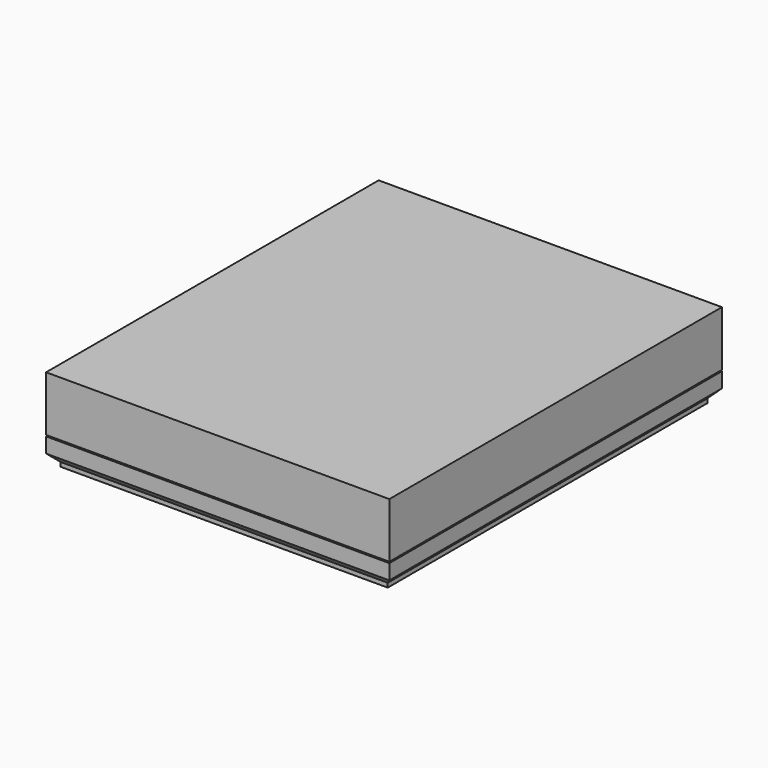
from build123d import *

# Parameters (mm, degrees)
F3_W          = 80.6
F3_H          = 97.6
F4_DEPTH      = 1
F5_W          = 80.6
F5_H          = 97.6
F5_W_2        = 73.6
F5_H_2        = 90.6
F6_DEPTH      = 8.75
F8_DEPTH      = 90.6
F11_W         = 80.6
F11_H         = 97.6
F11_W_2       = 76.8
F11_H_2       = 93.8
F13_DEPTH     = 3.3
F14_W         = 80.6
F14_H         = 97.6
F14_W_2       = 76.8
F14_H_2       = 93.8
F15_DEPTH     = 3
F16_T4_DEPTH  = 76.8
F16_T9_DEPTH  = 93.8
F16_T14_DEPTH = 76.8
F16_T19_DEPTH = 93.8
F16_T25_DEPTH = 81.9433659759
F16_T31_DEPTH = 98.9433659759
F16_T40_DEPTH = 81.9433659759
F16_T46_DEPTH = 98.9433659759
F16_T55_DEPTH = 81.9433659759
F16_T61_DEPTH = 98.9433659759
F16_T70_DEPTH = 98.9433659759
F16_T76_DEPTH = 81.9433659759
F17_W         = 80.6
F17_H         = 97.6
F17_W_2       = 77.4
F17_H_2       = 94.4
F18_DEPTH     = 3.2


# Not quite as in the source:
# - a fillet or chamfer that OpenCascade refuses, or shapes differently, is made with other operations: its cross-section is extruded or revolved along the edge and cut away or added


with BuildPart() as f4:
    # F3 (on Top) → F4 (new body)
    with BuildSketch(Plane.XY):
        Rectangle(F3_W, F3_H)
    extrude(amount=F4_DEPTH)

    # F5 (on face) → F6 (join)
    with BuildSketch(Plane.XY.offset(1)):
        Rectangle(F5_W, F5_H)
        Rectangle(F5_W_2, F5_H_2, mode=Mode.SUBTRACT)
    extrude(amount=F6_DEPTH)

    # F7 (on face) → F8 (join, through all)
    with BuildSketch(Plane.XZ.offset(-45.3)):
        with BuildLine():
            ThreePointArc((-19.9, 9.75), (-28.35, 1.3), (-36.8, 9.75))
            Line((-36.8, 9.75), (-36.8, 1))
            Line((-36.8, 1), (36.8, 1))
            Line((36.8, 1), (36.8, 9.75))
            ThreePointArc((36.8, 9.75), (28.35, 1.3), (19.9, 9.75))
            Line((19.9, 9.75), (17.9, 9.75))
            ThreePointArc((17.9, 9.75), (9.45, 1.3), (1, 9.75))
            Line((1, 9.75), (-1, 9.75))
            ThreePointArc((-1, 9.75), (-9.45, 1.3), (-17.9, 9.75))
            Line((-17.9, 9.75), (-19.9, 9.75))
        make_face()
    extrude(amount=F8_DEPTH)


with BuildPart() as f10_1:
    # F10: instance of F4
    add(f4.part.mirror(Plane.XY.offset(9.85)))

    # F17 (on face) → F18 (join)
    with BuildSketch(Plane(origin=(0, 0, 9.95), x_dir=(1, 0, 0), z_dir=(0, 0, -1))):
        Rectangle(F17_W, F17_H)
        Rectangle(F17_W_2, F17_H_2, mode=Mode.SUBTRACT)
    extrude(amount=F18_DEPTH)


with BuildPart() as f4_1:
    add(f4.part)

    # F11 (on face) → F13 (cut)
    with BuildSketch(Plane.XY.offset(9.75)):
        Rectangle(F11_W, F11_H)
        Rectangle(F11_W_2, F11_H_2, mode=Mode.SUBTRACT)
    extrude(amount=-F13_DEPTH, mode=Mode.SUBTRACT)

    # F14 (on face) → F15 (cut)
    with BuildSketch(Plane(origin=(0, 0, 0), x_dir=(1, 0, 0), z_dir=(0, 0, -1))):
        Rectangle(F14_W, F14_H)
        Rectangle(F14_W_2, F14_H_2, mode=Mode.SUBTRACT)
    extrude(amount=-F15_DEPTH, mode=Mode.SUBTRACT)

    # F16: chamfer of 2 on 4 edges, made by hand


with BuildPart() as f16_tool2:
    # F16_s3 → F16_t4 (new body)
    with BuildSketch(Plane.YZ.offset(-38.4)):
        Polygon((-48.9, 3), (-46.9, 1), (-46.9, 3), align=None)
    extrude(amount=F16_T4_DEPTH)

    split(bisect_by=Plane.XZ.offset(48.8), keep=Keep.BOTTOM)


with BuildPart() as f4_2:
    add(f4_1.part)

    # F16_t1: union F16_tool2
    add(f16_tool2.part)


with BuildPart() as f16_tool7:
    # F16_s8 → F16_t9 (new body)
    with BuildSketch(Plane.XZ.offset(-46.9)):
        Polygon((-40.4, 3), (-38.4, 1), (-38.4, 3), align=None)
    extrude(amount=F16_T9_DEPTH)

    split(bisect_by=Plane.YZ.offset(-40.3), keep=Keep.TOP)


with BuildPart() as f4_3:
    add(f4_2.part)

    # F16_t6: union F16_tool7
    add(f16_tool7.part)


with BuildPart() as f16_tool12:
    # F16_s13 → F16_t14 (new body)
    with BuildSketch(Plane.YZ.offset(38.4)):
        Polygon((48.9, 3), (46.9, 1), (46.9, 3), align=None)
    extrude(amount=-F16_T14_DEPTH)

    split(bisect_by=Plane.XZ.offset(-48.8), keep=Keep.TOP)


with BuildPart() as f4_4:
    add(f4_3.part)

    # F16_t11: union F16_tool12
    add(f16_tool12.part)


with BuildPart() as f16_tool17:
    # F16_s18 → F16_t19 (new body)
    with BuildSketch(Plane.XZ.offset(46.9)):
        Polygon((40.4, 3), (38.4, 1), (38.4, 3), align=None)
    extrude(amount=-F16_T19_DEPTH)

    split(bisect_by=Plane.YZ.offset(40.3), keep=Keep.BOTTOM)


with BuildPart() as f4_5:
    add(f4_4.part)

    # F16_t16: union F16_tool17
    add(f16_tool17.part)


with BuildPart() as f16_tool23:
    # F16_s24 → F16_t25 (new body)
    with BuildSketch(Plane.YZ.offset(-43.5433659759)):
        Polygon((-48.9, 3), (-46.9, 1), (-46.9, 3), align=None)
    extrude(amount=F16_T25_DEPTH)

    split(bisect_by=Plane.XZ.offset(48.8), keep=Keep.BOTTOM)

    split(bisect_by=Plane.YZ.offset(-40.3), keep=Keep.TOP)

    split(bisect_by=Plane.YZ.offset(-38.4), keep=Keep.BOTTOM)


with BuildPart() as f16_tool29:
    # F16_s30 → F16_t31 (new body)
    with BuildSketch(Plane.XZ.offset(-46.9)):
        Polygon((-40.4, 3), (-38.4, 1), (-38.4, 3), align=None)
    extrude(amount=F16_T31_DEPTH)

    split(bisect_by=Plane.XZ.offset(48.8), keep=Keep.BOTTOM)

    split(bisect_by=Plane.YZ.offset(-40.3), keep=Keep.TOP)

    split(bisect_by=Plane.XZ.offset(46.9), keep=Keep.TOP)


with BuildPart() as f16_tool23_1:
    add(f16_tool23.part)

    # F16_t35: intersect F16_tool29
    add(f16_tool29.part, mode=Mode.INTERSECT)


with BuildPart() as f4_6:
    add(f4_5.part)

    # F16_t21: union F16_tool23
    add(f16_tool23_1.part)


with BuildPart() as f16_tool38:
    # F16_s39 → F16_t40 (new body)
    with BuildSketch(Plane.YZ.offset(-38.4)):
        Polygon((-48.9, 3), (-46.9, 1), (-46.9, 3), align=None)
    extrude(amount=F16_T40_DEPTH)

    split(bisect_by=Plane.XZ.offset(48.8), keep=Keep.BOTTOM)

    split(bisect_by=Plane.YZ.offset(40.3), keep=Keep.BOTTOM)

    split(bisect_by=Plane.YZ.offset(38.4), keep=Keep.TOP)


with BuildPart() as f16_tool44:
    # F16_s45 → F16_t46 (new body)
    with BuildSketch(Plane.XZ.offset(52.0433659759)):
        Polygon((40.4, 3), (38.4, 1), (38.4, 3), align=None)
    extrude(amount=-F16_T46_DEPTH)

    split(bisect_by=Plane.XZ.offset(48.8), keep=Keep.BOTTOM)

    split(bisect_by=Plane.YZ.offset(40.3), keep=Keep.BOTTOM)

    split(bisect_by=Plane.XZ.offset(46.9), keep=Keep.TOP)


with BuildPart() as f16_tool38_1:
    add(f16_tool38.part)

    # F16_t50: intersect F16_tool44
    add(f16_tool44.part, mode=Mode.INTERSECT)


with BuildPart() as f4_7:
    add(f4_6.part)

    # F16_t36: union F16_tool38
    add(f16_tool38_1.part)


with BuildPart() as f16_tool53:
    # F16_s54 → F16_t55 (new body)
    with BuildSketch(Plane.YZ.offset(38.4)):
        Polygon((48.9, 3), (46.9, 1), (46.9, 3), align=None)
    extrude(amount=-F16_T55_DEPTH)

    split(bisect_by=Plane.YZ.offset(-40.3), keep=Keep.TOP)

    split(bisect_by=Plane.XZ.offset(-48.8), keep=Keep.TOP)

    split(bisect_by=Plane.YZ.offset(-38.4), keep=Keep.BOTTOM)


with BuildPart() as f16_tool59:
    # F16_s60 → F16_t61 (new body)
    with BuildSketch(Plane.XZ.offset(-52.0433659759)):
        Polygon((-40.4, 3), (-38.4, 1), (-38.4, 3), align=None)
    extrude(amount=F16_T61_DEPTH)

    split(bisect_by=Plane.YZ.offset(-40.3), keep=Keep.TOP)

    split(bisect_by=Plane.XZ.offset(-48.8), keep=Keep.TOP)

    split(bisect_by=Plane.XZ.offset(-46.9), keep=Keep.BOTTOM)


with BuildPart() as f16_tool53_1:
    add(f16_tool53.part)

    # F16_t65: intersect F16_tool59
    add(f16_tool59.part, mode=Mode.INTERSECT)


with BuildPart() as f4_8:
    add(f4_7.part)

    # F16_t51: union F16_tool53
    add(f16_tool53_1.part)


with BuildPart() as f16_tool68:
    # F16_s69 → F16_t70 (new body)
    with BuildSketch(Plane.XZ.offset(46.9)):
        Polygon((40.4, 3), (38.4, 1), (38.4, 3), align=None)
    extrude(amount=-F16_T70_DEPTH)

    split(bisect_by=Plane.YZ.offset(40.3), keep=Keep.BOTTOM)

    split(bisect_by=Plane.XZ.offset(-48.8), keep=Keep.TOP)

    split(bisect_by=Plane.XZ.offset(-46.9), keep=Keep.BOTTOM)


with BuildPart() as f16_tool74:
    # F16_s75 → F16_t76 (new body)
    with BuildSketch(Plane.YZ.offset(43.5433659759)):
        Polygon((48.9, 3), (46.9, 1), (46.9, 3), align=None)
    extrude(amount=-F16_T76_DEPTH)

    split(bisect_by=Plane.YZ.offset(40.3), keep=Keep.BOTTOM)

    split(bisect_by=Plane.XZ.offset(-48.8), keep=Keep.TOP)

    split(bisect_by=Plane.YZ.offset(38.4), keep=Keep.TOP)


with BuildPart() as f16_tool68_1:
    add(f16_tool68.part)

    # F16_t80: intersect F16_tool74
    add(f16_tool74.part, mode=Mode.INTERSECT)


with BuildPart() as f4_9:
    add(f4_8.part)

    # F16_t66: union F16_tool68
    add(f16_tool68_1.part)


solid = Compound([f10_1.part, f4_9.part])
